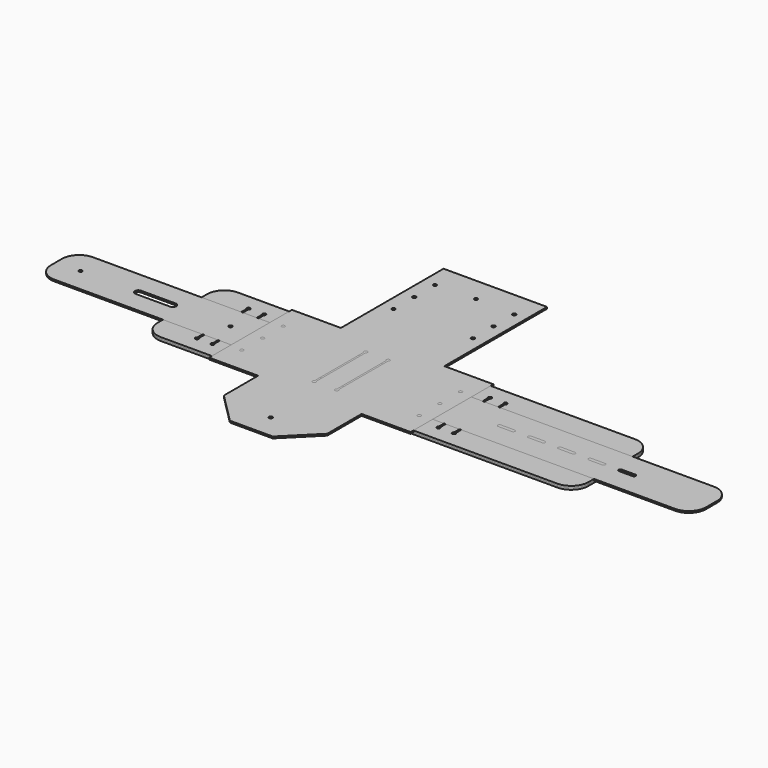
from build123d import *

# Parameters (mm, degrees)
F1_R     = 1
F4_DEPTH = 1
F2_R     = 1
F5_DEPTH = 1
F3_R     = 1
F6_DEPTH = 1
F7_R     = 1
F8_DEPTH = 1


# Not quite as in the source:
# - a feature names something its author has since deleted; it is built from what else it names


with BuildPart() as f4:
    # F1 (on Top) → F4 (new body)
    with BuildSketch(Plane.XY):
        with BuildLine():
            ThreePointArc((125, 18), (122.0710678119, 25.0710678119), (115, 28))
            Line((115, 28), (-115, 28))
            ThreePointArc((-115, 28), (-122.0710678119, 25.0710678119), (-125, 18))
            Line((-125, 18), (-125, -18))
            ThreePointArc((-125, -18), (-122.0710678119, -25.0710678119), (-115, -28))
            Line((-115, -28), (115, -28))
            ThreePointArc((115, -28), (122.0710678119, -25.0710678119), (125, -18))
            Line((125, -18), (125, 18))
        make_face()
        with BuildLine():
            ThreePointArc((115, 25), (119.9497474683, 22.9497474683), (122, 18))
            Line((122, 18), (122, -18))
            ThreePointArc((122, -18), (119.9497474683, -22.9497474683), (115, -25))
            Line((115, -25), (-115, -25))
            ThreePointArc((-115, -25), (-119.9497474683, -22.9497474683), (-122, -18))
            Line((-122, -18), (-122, 18))
            ThreePointArc((-122, 18), (-119.9497474683, 22.9497474683), (-115, 25))
            Line((-115, 25), (115, 25))
        make_face(mode=Mode.SUBTRACT)
        with BuildLine():
            Line((122, -18), (122, 18))
            ThreePointArc((122, 18), (119.9497474683, 22.9497474683), (115, 25))
            Line((115, 25), (-115, 25))
            ThreePointArc((-115, 25), (-119.9497474683, 22.9497474683), (-122, 18))
            Line((-122, 18), (-122, -18))
            ThreePointArc((-122, -18), (-119.9497474683, -22.9497474683), (-115, -25))
            Line((-115, -25), (115, -25))
            ThreePointArc((115, -25), (119.9497474683, -22.9497474683), (122, -18))
        make_face()
        with Locations((-97, 0)):
            Circle(F1_R, mode=Mode.SUBTRACT)
        with Locations((-69, 0)):
            Circle(F1_R, mode=Mode.SUBTRACT)
    extrude(amount=-F4_DEPTH)


with BuildPart() as f5:
    # F2 (on Top) → F5 (new body)
    with BuildSketch(Plane.XY):
        with BuildLine():
            ThreePointArc((125, 18), (122.0710678119, 25.0710678119), (115, 28))
            Line((115, 28), (-115, 28))
            ThreePointArc((-115, 28), (-122.0710678119, 25.0710678119), (-125, 18))
            Line((-125, 18), (-125, -18))
            ThreePointArc((-125, -18), (-122.0710678119, -25.0710678119), (-115, -28))
            Line((-115, -28), (115, -28))
            ThreePointArc((115, -28), (122.0710678119, -25.0710678119), (125, -18))
            Line((125, -18), (125, 18))
        make_face()
        with BuildLine():
            Line((-115, 25), (115, 25))
            ThreePointArc((115, 25), (119.9497474683, 22.9497474683), (122, 18))
            Line((122, 18), (122, -18))
            ThreePointArc((122, -18), (119.9497474683, -22.9497474683), (115, -25))
            Line((115, -25), (-115, -25))
            ThreePointArc((-115, -25), (-119.9497474683, -22.9497474683), (-122, -18))
            Line((-122, -18), (-122, 18))
            ThreePointArc((-122, 18), (-119.9497474683, 22.9497474683), (-115, 25))
        make_face(mode=Mode.SUBTRACT)
        with BuildLine():
            ThreePointArc((122, 18), (119.9497474683, 22.9497474683), (115, 25))
            Line((115, 25), (-115, 25))
            ThreePointArc((-115, 25), (-119.9497474683, 22.9497474683), (-122, 18))
            Line((-122, 18), (-122, -18))
            ThreePointArc((-122, -18), (-119.9497474683, -22.9497474683), (-115, -25))
            Line((-115, -25), (115, -25))
            ThreePointArc((115, -25), (119.9497474683, -22.9497474683), (122, -18))
            Line((122, -18), (122, 18))
        make_face()
        with BuildLine():
            Line((-102, -17.8006412629), (-102, 17.8006412629))
            ThreePointArc((-102, 17.8006412629), (-102, 19.5326920705), (-100.5, 18.6666666667))
            ThreePointArc((-100.5, 18.6666666667), (-100.6339745962, 18.1666666667), (-101, 17.8006412629))
            Line((-101, 17.8006412629), (-101, -17.8006412629))
            ThreePointArc((-101, -17.8006412629), (-100.6339745962, -18.1666666667), (-100.5, -18.6666666667))
            ThreePointArc((-100.5, -18.6666666667), (-102, -19.5326920705), (-102, -17.8006412629))
        make_face(mode=Mode.SUBTRACT)
        with Locations((-97, 0)):
            Circle(F2_R, mode=Mode.SUBTRACT)
        with BuildLine():
            Line((-92, 17.8006412629), (-92, -17.8006412629))
            ThreePointArc((-92, -17.8006412629), (-91.6339745962, -18.1666666667), (-91.5, -18.6666666667))
            ThreePointArc((-91.5, -18.6666666667), (-93, -19.5326920705), (-93, -17.8006412629))
            Line((-93, -17.8006412629), (-93, 17.8006412629))
            ThreePointArc((-93, 17.8006412629), (-93, 19.5326920705), (-91.5, 18.6666666667))
            ThreePointArc((-91.5, 18.6666666667), (-91.6339745962, 18.1666666667), (-92, 17.8006412629))
        make_face(mode=Mode.SUBTRACT)
        with BuildLine():
            Line((-74, -17.8006412629), (-74, 17.8006412629))
            ThreePointArc((-74, 17.8006412629), (-74, 19.5326920705), (-72.5, 18.6666666667))
            ThreePointArc((-72.5, 18.6666666667), (-72.6339745962, 18.1666666667), (-73, 17.8006412629))
            Line((-73, 17.8006412629), (-73, -17.8006412629))
            ThreePointArc((-73, -17.8006412629), (-72.6339745962, -18.1666666667), (-72.5, -18.6666666667))
            ThreePointArc((-72.5, -18.6666666667), (-74, -19.5326920705), (-74, -17.8006412629))
        make_face(mode=Mode.SUBTRACT)
        with Locations((-69, 0)):
            Circle(F2_R, mode=Mode.SUBTRACT)
        with BuildLine():
            Line((-64, 17.8006412629), (-64, -17.8006412629))
            ThreePointArc((-64, -17.8006412629), (-63.6339745962, -18.1666666667), (-63.5, -18.6666666667))
            ThreePointArc((-63.5, -18.6666666667), (-65, -19.5326920705), (-65, -17.8006412629))
            Line((-65, -17.8006412629), (-65, 17.8006412629))
            ThreePointArc((-65, 17.8006412629), (-65, 19.5326920705), (-63.5, 18.6666666667))
            ThreePointArc((-63.5, 18.6666666667), (-63.6339745962, 18.1666666667), (-64, 17.8006412629))
        make_face(mode=Mode.SUBTRACT)
        with BuildLine():
            Line((-46, -17.8006412629), (-46, 17.8006412629))
            ThreePointArc((-46, 17.8006412629), (-46, 19.5326920705), (-44.5, 18.6666666667))
            ThreePointArc((-44.5, 18.6666666667), (-44.6339745962, 18.1666666667), (-45, 17.8006412629))
            Line((-45, 17.8006412629), (-45, -17.8006412629))
            ThreePointArc((-45, -17.8006412629), (-44.6339745962, -18.1666666667), (-44.5, -18.6666666667))
            ThreePointArc((-44.5, -18.6666666667), (-46, -19.5326920705), (-46, -17.8006412629))
        make_face(mode=Mode.SUBTRACT)
        with BuildLine():
            Line((-36, 17.8006412629), (-36, -17.8006412629))
            ThreePointArc((-36, -17.8006412629), (-35.6339745962, -18.1666666667), (-35.5, -18.6666666667))
            ThreePointArc((-35.5, -18.6666666667), (-37, -19.5326920705), (-37, -17.8006412629))
            Line((-37, -17.8006412629), (-37, 17.8006412629))
            ThreePointArc((-37, 17.8006412629), (-37, 19.5326920705), (-35.5, 18.6666666667))
            ThreePointArc((-35.5, 18.6666666667), (-35.6339745962, 18.1666666667), (-36, 17.8006412629))
        make_face(mode=Mode.SUBTRACT)
        with BuildLine():
            Line((-17, 17.8006412629), (-17, -17.8006412629))
            ThreePointArc((-17, -17.8006412629), (-16.6339745962, -18.1666666667), (-16.5, -18.6666666667))
            ThreePointArc((-16.5, -18.6666666667), (-18, -19.5326920705), (-18, -17.8006412629))
            Line((-18, -17.8006412629), (-18, 17.8006412629))
            ThreePointArc((-18, 17.8006412629), (-18, 19.5326920705), (-16.5, 18.6666666667))
            ThreePointArc((-16.5, 18.6666666667), (-16.6339745962, 18.1666666667), (-17, 17.8006412629))
        make_face(mode=Mode.SUBTRACT)
        with BuildLine():
            Line((-9, -17.8006412629), (-9, 17.8006412629))
            ThreePointArc((-9, 17.8006412629), (-9, 19.5326920705), (-7.5, 18.6666666667))
            ThreePointArc((-7.5, 18.6666666667), (-7.6339745962, 18.1666666667), (-8, 17.8006412629))
            Line((-8, 17.8006412629), (-8, -17.8006412629))
            ThreePointArc((-8, -17.8006412629), (-7.6339745962, -18.1666666667), (-7.5, -18.6666666667))
            ThreePointArc((-7.5, -18.6666666667), (-9, -19.5326920705), (-9, -17.8006412629))
        make_face(mode=Mode.SUBTRACT)
        with BuildLine():
            Line((10, -17.8006412629), (10, 17.8006412629))
            ThreePointArc((10, 17.8006412629), (10, 19.5326920705), (11.5, 18.6666666667))
            ThreePointArc((11.5, 18.6666666667), (11.3660254038, 18.1666666667), (11, 17.8006412629))
            Line((11, 17.8006412629), (11, -17.8006412629))
            ThreePointArc((11, -17.8006412629), (11.3660254038, -18.1666666667), (11.5, -18.6666666667))
            ThreePointArc((11.5, -18.6666666667), (10, -19.5326920705), (10, -17.8006412629))
        make_face(mode=Mode.SUBTRACT)
        with BuildLine():
            Line((20, 17.8006412629), (20, -17.8006412629))
            ThreePointArc((20, -17.8006412629), (20.3660254038, -18.1666666667), (20.5, -18.6666666667))
            ThreePointArc((20.5, -18.6666666667), (19, -19.5326920705), (19, -17.8006412629))
            Line((19, -17.8006412629), (19, 17.8006412629))
            ThreePointArc((19, 17.8006412629), (19, 19.5326920705), (20.5, 18.6666666667))
            ThreePointArc((20.5, 18.6666666667), (20.3660254038, 18.1666666667), (20, 17.8006412629))
        make_face(mode=Mode.SUBTRACT)
        with BuildLine():
            Line((38, -17.8006412629), (38, 17.8006412629))
            ThreePointArc((38, 17.8006412629), (38, 19.5326920705), (39.5, 18.6666666667))
            ThreePointArc((39.5, 18.6666666667), (39.3660254038, 18.1666666667), (39, 17.8006412629))
            Line((39, 17.8006412629), (39, -17.8006412629))
            ThreePointArc((39, -17.8006412629), (39.3660254038, -18.1666666667), (39.5, -18.6666666667))
            ThreePointArc((39.5, -18.6666666667), (38, -19.5326920705), (38, -17.8006412629))
        make_face(mode=Mode.SUBTRACT)
        with BuildLine():
            Line((48, 17.8006412629), (48, -17.8006412629))
            ThreePointArc((48, -17.8006412629), (48.3660254038, -18.1666666667), (48.5, -18.6666666667))
            ThreePointArc((48.5, -18.6666666667), (47, -19.5326920705), (47, -17.8006412629))
            Line((47, -17.8006412629), (47, 17.8006412629))
            ThreePointArc((47, 17.8006412629), (47, 19.5326920705), (48.5, 18.6666666667))
            ThreePointArc((48.5, 18.6666666667), (48.3660254038, 18.1666666667), (48, 17.8006412629))
        make_face(mode=Mode.SUBTRACT)
    extrude(amount=F5_DEPTH)


with BuildPart() as f6:
    # F3 (on Top) → F6 (new body)
    with BuildSketch(Plane.XY):
        with BuildLine():
            ThreePointArc((-188, 14), (-195.0710678119, 11.0710678119), (-198, 4))
            Line((-198, 4), (-198, -4))
            ThreePointArc((-198, -4), (-195.0710678119, -11.0710678119), (-188, -14))
            Line((-188, -14), (172, -14))
            ThreePointArc((172, -14), (179.0710678119, -11.0710678119), (182, -4))
            Line((182, -4), (182, 4))
            ThreePointArc((182, 4), (179.0710678119, 11.0710678119), (172, 14))
            Line((172, 14), (-188, 14))
        make_face()
        with BuildLine():
            ThreePointArc((172, 12), (177.6568542495, 9.6568542495), (180, 4))
            Line((180, 4), (180, -4))
            ThreePointArc((180, -4), (177.6568542495, -9.6568542495), (172, -12))
            Line((172, -12), (-188, -12))
            ThreePointArc((-188, -12), (-193.6568542495, -9.6568542495), (-196, -4))
            Line((-196, -4), (-196, 4))
            ThreePointArc((-196, 4), (-194.164414003, 9.0990195136), (-189.5, 11.8581168228))
            Line((-189.5, 11.8581168228), (-189.5, 12.375))
            Line((-189.5, 12.375), (-186.5, 12.375))
            Line((-186.5, 12.375), (-186.5, 12))
            Line((-186.5, 12), (172, 12))
        make_face(mode=Mode.SUBTRACT)
        with BuildLine():
            Line((180, -4), (180, 4))
            ThreePointArc((180, 4), (177.6568542495, 9.6568542495), (172, 12))
            Line((172, 12), (-186.5, 12))
            Line((-186.5, 12), (-186.5, 11.625))
            Line((-186.5, 11.625), (-189.5, 11.625))
            Line((-189.5, 11.625), (-189.5, 11.8581168228))
            ThreePointArc((-189.5, 11.8581168228), (-194.164414003, 9.0990195136), (-196, 4))
            Line((-196, 4), (-196, -4))
            ThreePointArc((-196, -4), (-193.6568542495, -9.6568542495), (-188, -12))
            Line((-188, -12), (172, -12))
            ThreePointArc((172, -12), (177.6568542495, -9.6568542495), (180, -4))
        make_face()
        with Locations((-184, 0)):
            Circle(F3_R, mode=Mode.SUBTRACT)
        with BuildLine():
            Line((-130.5, -2), (-150.5, -2))
            ThreePointArc((-150.5, -2), (-152.5, 0), (-150.5, 2))
            Line((-150.5, 2), (-130.5, 2))
            ThreePointArc((-130.5, 2), (-128.5, 0), (-130.5, -2))
        make_face(mode=Mode.SUBTRACT)
        with Locations((-97, 0)):
            Circle(F3_R, mode=Mode.SUBTRACT)
        with Locations((-69, 0)):
            Circle(F3_R, mode=Mode.SUBTRACT)
        with BuildLine():
            Line((59, 1), (67, 1))
            ThreePointArc((67, 1), (68, 0), (67, -1))
            Line((67, -1), (59, -1))
            ThreePointArc((59, -1), (58, 0), (59, 1))
        make_face(mode=Mode.SUBTRACT)
        with BuildLine():
            Line((84.5, -1), (76.5, -1))
            ThreePointArc((76.5, -1), (75.5, 0), (76.5, 1))
            Line((76.5, 1), (84.5, 1))
            ThreePointArc((84.5, 1), (85.5, 0), (84.5, -1))
        make_face(mode=Mode.SUBTRACT)
        with BuildLine():
            Line((102, -1), (94, -1))
            ThreePointArc((94, -1), (93, 0), (94, 1))
            Line((94, 1), (102, 1))
            ThreePointArc((102, 1), (103, 0), (102, -1))
        make_face(mode=Mode.SUBTRACT)
        with BuildLine():
            Line((111.5, 1), (119.5, 1))
            ThreePointArc((119.5, 1), (120.5, 0), (119.5, -1))
            Line((119.5, -1), (111.5, -1))
            ThreePointArc((111.5, -1), (110.5, 0), (111.5, 1))
        make_face(mode=Mode.SUBTRACT)
        with BuildLine():
            Line((129, 1), (137, 1))
            ThreePointArc((137, 1), (138, 0), (137, -1))
            Line((137, -1), (129, -1))
            ThreePointArc((129, -1), (128, 0), (129, 1))
        make_face(mode=Mode.SUBTRACT)
        with BuildLine():
            Line((-188, 12), (-186.5, 12))
            Line((-186.5, 12), (-186.5, 12.375))
            Line((-186.5, 12.375), (-189.5, 12.375))
            Line((-189.5, 12.375), (-189.5, 11.8581168228))
            ThreePointArc((-189.5, 11.8581168228), (-188.7533476681, 11.964450219), (-188, 12))
        make_face()
        with BuildLine():
            Line((-186.5, 11.625), (-186.5, 12))
            Line((-186.5, 12), (-188, 12))
            ThreePointArc((-188, 12), (-188.7533476681, 11.964450219), (-189.5, 11.8581168228))
            Line((-189.5, 11.8581168228), (-189.5, 11.625))
            Line((-189.5, 11.625), (-186.5, 11.625))
        make_face()
    extrude(amount=F6_DEPTH)


with BuildPart() as f8:
    # F7 (on Top) → F8 (new body)
    with BuildSketch(Plane.XY):
        Polygon((-85.4247779608, -30), (-57, -30), (-57, -54.851184832), (-39.4264068712, -72.4247779608), (-14.5735931288, -72.4247779608), (3, -54.851184832), (3, -30), (31.4247779608, -30), (31.4247779608, 30), (3, 30), (3, 104.4247779608), (-57, 104.4247779608), (-57, 30), (-85.4247779608, 30), align=None)
        with Locations((-27, -58.4247779608)):
            Circle(F7_R, mode=Mode.SUBTRACT)
        with Locations((-78.4247779608, -15)):
            Circle(F7_R, mode=Mode.SUBTRACT)
        with Locations((-78.4247779608, 0)):
            Circle(F7_R, mode=Mode.SUBTRACT)
        with Locations((-78.4247779608, 15)):
            Circle(F7_R, mode=Mode.SUBTRACT)
        with BuildLine():
            Line((-33, 17.8006412629), (-33, -17.8006412629))
            ThreePointArc((-33, -17.8006412629), (-32.6339745962, -18.1666666667), (-32.5, -18.6666666667))
            ThreePointArc((-32.5, -18.6666666667), (-34, -19.5326920705), (-34, -17.8006412629))
            Line((-34, -17.8006412629), (-34, 17.8006412629))
            ThreePointArc((-34, 17.8006412629), (-34, 19.5326920705), (-32.5, 18.6666666667))
            ThreePointArc((-32.5, 18.6666666667), (-32.6339745962, 18.1666666667), (-33, 17.8006412629))
        make_face(mode=Mode.SUBTRACT)
        with BuildLine():
            Line((-21, -17.8006412629), (-21, 17.8006412629))
            ThreePointArc((-21, 17.8006412629), (-21, 19.5326920705), (-19.5, 18.6666666667))
            ThreePointArc((-19.5, 18.6666666667), (-19.6339745962, 18.1666666667), (-20, 17.8006412629))
            Line((-20, 17.8006412629), (-20, -17.8006412629))
            ThreePointArc((-20, -17.8006412629), (-19.6339745962, -18.1666666667), (-19.5, -18.6666666667))
            ThreePointArc((-19.5, -18.6666666667), (-21, -19.5326920705), (-21, -17.8006412629))
        make_face(mode=Mode.SUBTRACT)
        with Locations((24.4247779608, -15)):
            Circle(F7_R, mode=Mode.SUBTRACT)
        with Locations((24.4247779608, 0)):
            Circle(F7_R, mode=Mode.SUBTRACT)
        with Locations((24.4247779608, 15)):
            Circle(F7_R, mode=Mode.SUBTRACT)
        with Locations((-50, 59.4247779608)):
            Circle(F7_R, mode=Mode.SUBTRACT)
        with Locations((-50, 74.4247779608)):
            Circle(F7_R, mode=Mode.SUBTRACT)
        with Locations((-50, 89.4247779608)):
            Circle(F7_R, mode=Mode.SUBTRACT)
        with Locations((-27, 90.4247779608)):
            Circle(F7_R, mode=Mode.SUBTRACT)
        with Locations((-4, 59.4247779608)):
            Circle(F7_R, mode=Mode.SUBTRACT)
        with Locations((-4, 74.4247779608)):
            Circle(F7_R, mode=Mode.SUBTRACT)
        with Locations((-4, 89.4247779608)):
            Circle(F7_R, mode=Mode.SUBTRACT)
    extrude(amount=F8_DEPTH)


solid = Compound([f4.part, f5.part, f6.part, f8.part])
